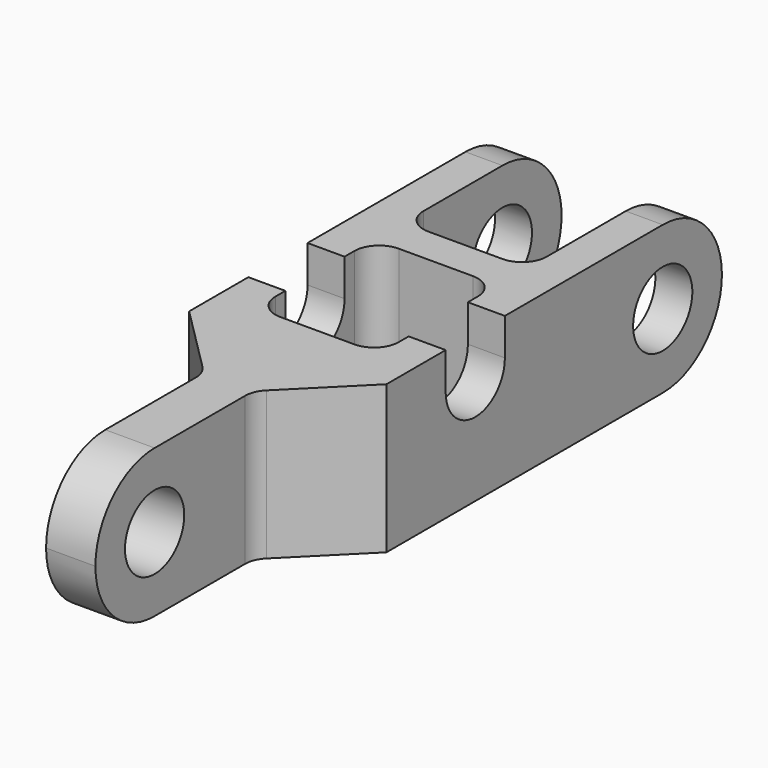
from build123d import *

# Parameters (mm, degrees)
F1_DEPTH = 9.525
F2_R     = 1.5875
F3_R     = 4.76249
F4_R     = 2.38125
F5_DEPTH = 12.7


# Not quite as in the source:
# - a fillet or chamfer is up to 0.001 mm smaller than in the source, because OpenCascade refuses the exact size


with BuildPart() as f1:
    # F0 (on Top) → F1 (new body)
    with BuildSketch(Plane.XY):
        Polygon((0, 12.7), (0, 0), (3.175, 0), (3.175, 12.7), (7.9375, 17.4625), (7.9375, 44.45), (5.55625, 44.45), (5.55625, 31.75), (1.5875, 31.75), (-2.38125, 31.75), (-2.38125, 44.45), (-4.7625, 44.45), (-4.7625, 17.4625), align=None)
        Polygon((-2.38125, 29.36875), (1.5875, 29.36875), (5.55625, 29.36875), (5.55625, 19.84375), (-2.38125, 19.84375), align=None, mode=Mode.SUBTRACT)
    extrude(amount=F1_DEPTH)

    # F2
    f2_edges = [f1.edges().sort_by_distance(p)[0] for p in [
        (-2.38125, 31.75, 4.7625),
        (5.55625, 31.75, 4.7625),
        (5.55625, 29.36875, 4.7625),
        (-2.38125, 29.36875, 4.7625),
        (-2.38125, 19.84375, 4.7625),
        (5.55625, 19.84375, 4.7625),
        (0, 12.7, 4.7625),
        (3.175, 12.7, 4.7625),
    ]]
    fillet(f2_edges, radius=F2_R)

    # F3 (radius 4.7625 in the source; OpenCascade refuses exactly that, so slightly less here)
    f3_edges = [f1.edges().sort_by_distance(p)[0] for p in [
        (1.5875, 0, 9.525),
        (1.5875, 0, 0),
        (-3.571875, 44.45, 9.525),
        (-3.571875, 44.45, 0),
        (6.746875, 44.45, 9.525),
        (6.746875, 44.45, 0),
    ]]
    fillet(f3_edges, radius=F3_R)

    # F4 (on face) → F5 (cut, through all)
    with BuildSketch(Plane(origin=(-4.7625, 0, 0), x_dir=(0, -1, 0), z_dir=(-1, 0, 0))):
        with Locations((-39.6875, 4.7625)):
            Circle(F4_R)
        with Locations((-4.7625, 4.7625)):
            Circle(F4_R)
        with BuildLine():
            Line((-22.225, 9.525), (-26.9875, 9.525))
            Line((-26.9875, 9.525), (-26.9875, 7.14375))
            ThreePointArc((-26.9875, 7.14375), (-24.60625, 4.7625), (-22.225, 7.14375))
            Line((-22.225, 7.14375), (-22.225, 9.525))
        make_face()
    extrude(amount=-F5_DEPTH, mode=Mode.SUBTRACT)


solid = f1.part
